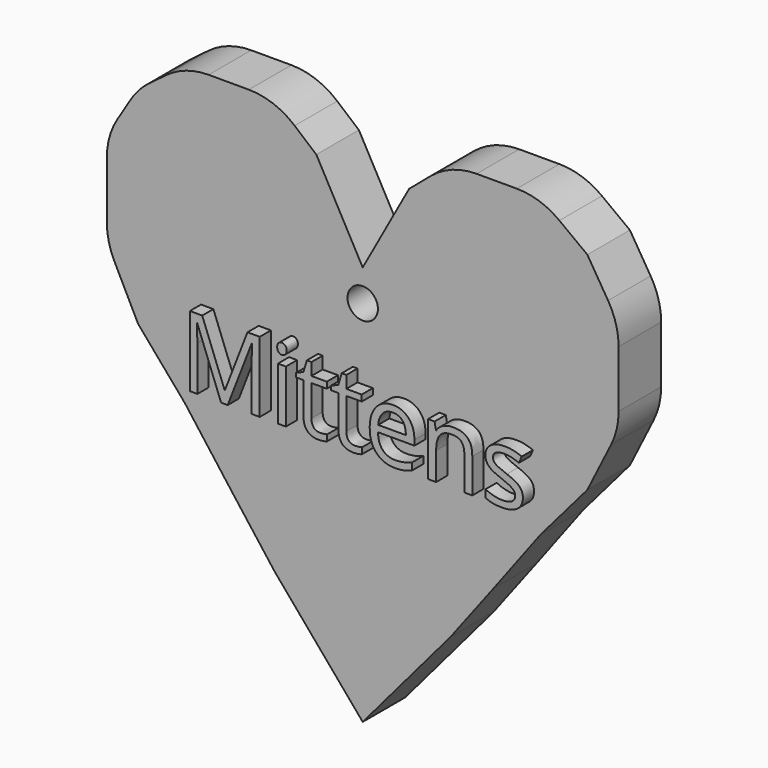
from build123d import *

# Parameters (mm, degrees)
F0_R         = 1.0891736151
F1_DEPTH     = 3.81
F2_TEXT_SIZE = 7.0771408351
F3_DEPTH     = 1
F4_TEXT_SIZE = 2.4694444444
F5_DEPTH     = 0.3048
F6_R         = 5.08
F7_R         = 5.08
F8_R         = 5.08
F9_R         = 5.08
F10_R        = 5.08
F11_R        = 5.08
F12_R        = 5.08
F13_R        = 5.08


# Not quite as in the source:
# - Text() gives the source's letters only with a copy of the font that has no kerning and outlines rounded to 1/6400 em; it was checked with that copy


with BuildPart() as f1:
    # F0 (on Front) → F1 (new body)
    with BuildSketch(Plane.XZ):
        Polygon((3.3220950087, 27.2761378437), (0, 21.2356609444), (-3.3220950087, 27.2761378437), (-6.2944935635, 29.7939348966), (-9.3718012795, 29.7939348966), (-12.7288633958, 29.7939348966), (-16.085928306, 27.2761378437), (-18.3239709586, 23.6393176019), (-18.3239709586, 19.7227448225), (-18.3239709586, 16.9251933694), (-16.085928306, 12.4491089955), (-12.7288633958, 8.5325352848), (-9.3718012795, 4.0564509109), (-6.2944935635, 0), (0, -7.4135139585), (6.2944935635, 0), (9.3718012795, 4.0564509109), (12.7288633958, 8.5325352848), (16.085928306, 12.4491089955), (18.3239709586, 16.9251933694), (18.3239709586, 19.7227448225), (18.3239709586, 23.6393176019), (16.085928306, 27.2761378437), (12.7288633958, 29.7939348966), (9.3718012795, 29.7939348966), (6.2944935635, 29.7939348966), align=None)
        with Locations((0, 18.9754962921)):
            Circle(F0_R, mode=Mode.SUBTRACT)
    extrude(amount=-F1_DEPTH)

    # F4 (on face) → F5 (cut)
    with BuildSketch(Plane(origin=(0, 3.81, 0), x_dir=(-1, 0, 0), z_dir=(0, 1, 0))):
        with Locations((-9.9481955295, 12.9554586574)):
            Text('40 Marsten Ln', F4_TEXT_SIZE, font='Open Sans', text_align=(TextAlign.LEFT, TextAlign.BOTTOM))
        with Locations((-9.9481955295, 9.5970142129)):
            Text('unit 114', F4_TEXT_SIZE, font='Open Sans', text_align=(TextAlign.LEFT, TextAlign.BOTTOM))
        with Locations((-9.9481955295, 6.2385697685)):
            Text('Enfield,NH 03748', F4_TEXT_SIZE, font='Open Sans', text_align=(TextAlign.LEFT, TextAlign.BOTTOM))
    extrude(amount=F5_DEPTH, mode=Mode.SUBTRACT)

    # F6
    f6_edges = [f1.edges().sort_by_distance(p)[0] for p in [
        (12.728863, 1.905, 29.793935),
        (6.294494, 1.905, 29.793935),
    ]]
    fillet(f6_edges, radius=F6_R)

    # F7
    f7_edges = [f1.edges().sort_by_distance(p)[0] for p in [
        (18.323971, 1.905, 23.639318),
    ]]
    fillet(f7_edges, radius=F7_R)

    # F8
    f8_edges = [f1.edges().sort_by_distance(p)[0] for p in [
        (18.323971, 1.905, 16.925193),
    ]]
    fillet(f8_edges, radius=F8_R)

    # F9
    f9_edges = [f1.edges().sort_by_distance(p)[0] for p in [
        (-6.294494, 1.905, 29.793935),
    ]]
    fillet(f9_edges, radius=F9_R)

    # F10
    f10_edges = [f1.edges().sort_by_distance(p)[0] for p in [
        (-12.728863, 1.905, 29.793935),
    ]]
    fillet(f10_edges, radius=F10_R)

    # F11
    f11_edges = [f1.edges().sort_by_distance(p)[0] for p in [
        (-16.085928, 1.905, 27.276138),
    ]]
    fillet(f11_edges, radius=F11_R)

    # F12
    f12_edges = [f1.edges().sort_by_distance(p)[0] for p in [
        (-18.323971, 1.905, 23.639318),
    ]]
    fillet(f12_edges, radius=F12_R)

    # F13
    f13_edges = [f1.edges().sort_by_distance(p)[0] for p in [
        (-18.323971, 1.905, 16.925193),
    ]]
    fillet(f13_edges, radius=F13_R)


with BuildPart() as f3:
    # F2 (on face) → F3 (new body)
    with BuildSketch(Plane.XZ):
        with Locations((-12.273255003, 10.0815141368)):
            Text('Mittens', F2_TEXT_SIZE, font='Open Sans', text_align=(TextAlign.LEFT, TextAlign.BOTTOM))
    extrude(amount=F3_DEPTH)


solid = Compound([f1.part, f3.part])
